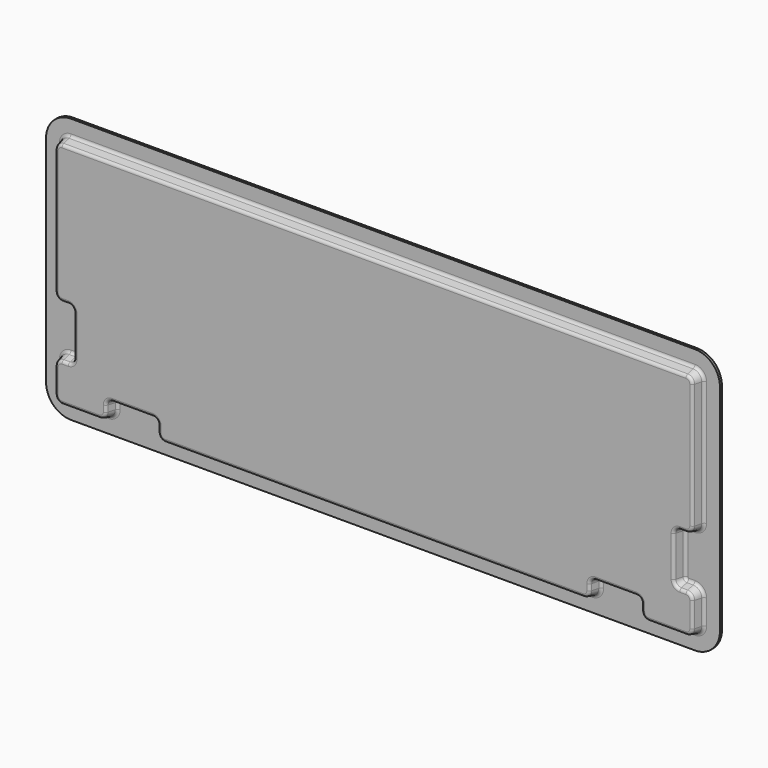
from build123d import *

# Parameters (mm, degrees)
F3_DEPTH = 2
F4_DEPTH = 18
F4_TAPER = -15
F5_R     = 5
F6_T     = 2
F7_DEPTH = 2


# Not quite as in the source:
# - a shell that OpenCascade refuses in one call is made with other operations: the cavity is built on its own and cut out


with BuildPart() as f3:
    # F0 (on Front) → F3 (new body)
    with BuildSketch(Plane.XZ):
        with BuildLine():
            ThreePointArc((540, 172.5), (528.2842712475, 200.7842712475), (500, 212.5))
            Line((500, 212.5), (-500, 212.5))
            ThreePointArc((-500, 212.5), (-528.2842712475, 200.7842712475), (-540, 172.5))
            Line((-540, 172.5), (-540, -172.5))
            ThreePointArc((-540, -172.5), (-528.2842712475, -200.7842712475), (-500, -212.5))
            Line((-500, -212.5), (500, -212.5))
            ThreePointArc((500, -212.5), (528.2842712475, -200.7842712475), (540, -172.5))
            Line((540, -172.5), (540, 172.5))
        make_face()
        with BuildLine():
            ThreePointArc((-525, 172.5), (-517.6776695297, 190.1776695297), (-500, 197.5))
            Line((-500, 197.5), (500, 197.5))
            ThreePointArc((500, 197.5), (517.6776695297, 190.1776695297), (525, 172.5))
            Line((525, 172.5), (525, -172.5))
            ThreePointArc((525, -172.5), (517.6776695297, -190.1776695297), (500, -197.5))
            Line((500, -197.5), (-500, -197.5))
            ThreePointArc((-500, -197.5), (-517.6776695297, -190.1776695297), (-525, -172.5))
            Line((-525, -172.5), (-525, 172.5))
        make_face(mode=Mode.SUBTRACT)
        with BuildLine():
            Line((500, 197.5), (-500, 197.5))
            ThreePointArc((-500, 197.5), (-517.6776695297, 190.1776695297), (-525, 172.5))
            Line((-525, 172.5), (-525, -172.5))
            ThreePointArc((-525, -172.5), (-517.6776695297, -190.1776695297), (-500, -197.5))
            Line((-500, -197.5), (500, -197.5))
            ThreePointArc((500, -197.5), (517.6776695297, -190.1776695297), (525, -172.5))
            Line((525, -172.5), (525, 172.5))
            ThreePointArc((525, 172.5), (517.6776695297, 190.1776695297), (500, 197.5))
        make_face()
    extrude(amount=F3_DEPTH)

    # F2 (on offset) → F4 (join, through all)
    with BuildSketch(Plane.XZ.offset(20)):
        with BuildLine():
            Line((510, -27.5), (510, 172.5))
            ThreePointArc((510, 172.5), (507.0710678119, 179.5710678119), (500, 182.5))
            Line((500, 182.5), (-500, 182.5))
            ThreePointArc((-500, 182.5), (-507.0710678119, 179.5710678119), (-510, 172.5))
            Line((-510, 172.5), (-510, -27.5))
            ThreePointArc((-510, -27.5), (-507.0710678119, -34.5710678119), (-500, -37.5))
            Line((-500, -37.5), (-490, -37.5))
            ThreePointArc((-490, -37.5), (-482.9289321881, -40.4289321881), (-480, -47.5))
            Line((-480, -47.5), (-480, -112.5))
            ThreePointArc((-480, -112.5), (-482.9289321881, -119.5710678119), (-490, -122.5))
            Line((-490, -122.5), (-500, -122.5))
            ThreePointArc((-500, -122.5), (-507.0710678119, -125.4289321881), (-510, -132.5))
            Line((-510, -132.5), (-510, -172.5))
            ThreePointArc((-510, -172.5), (-507.0710678119, -179.5710678119), (-500, -182.5))
            Line((-500, -182.5), (-440, -182.5))
            ThreePointArc((-440, -182.5), (-432.9289321881, -179.5710678119), (-430, -172.5))
            Line((-430, -172.5), (-430, -162.5))
            ThreePointArc((-430, -162.5), (-427.0710678119, -155.4289321881), (-420, -152.5))
            Line((-420, -152.5), (-355, -152.5))
            ThreePointArc((-355, -152.5), (-347.9289321881, -155.4289321881), (-345, -162.5))
            Line((-345, -162.5), (-345, -172.5))
            ThreePointArc((-345, -172.5), (-342.0710678119, -179.5710678119), (-335, -182.5))
            Line((-335, -182.5), (0, -182.5))
            Line((0, -182.5), (335, -182.5))
            ThreePointArc((335, -182.5), (342.0710678119, -179.5710678119), (345, -172.5))
            Line((345, -172.5), (345, -162.5))
            ThreePointArc((345, -162.5), (347.9289321881, -155.4289321881), (355, -152.5))
            Line((355, -152.5), (420, -152.5))
            ThreePointArc((420, -152.5), (427.0710678119, -155.4289321881), (430, -162.5))
            Line((430, -162.5), (430, -172.5))
            ThreePointArc((430, -172.5), (432.9289321881, -179.5710678119), (440, -182.5))
            Line((440, -182.5), (500, -182.5))
            ThreePointArc((500, -182.5), (507.0710678119, -179.5710678119), (510, -172.5))
            Line((510, -172.5), (510, -132.5))
            ThreePointArc((510, -132.5), (507.0710678119, -125.4289321881), (500, -122.5))
            Line((500, -122.5), (490, -122.5))
            ThreePointArc((490, -122.5), (482.9289321881, -119.5710678119), (480, -112.5))
            Line((480, -112.5), (480, -47.5))
            ThreePointArc((480, -47.5), (482.9289321881, -40.4289321881), (490, -37.5))
            Line((490, -37.5), (500, -37.5))
            ThreePointArc((500, -37.5), (507.0710678119, -34.5710678119), (510, -27.5))
        make_face()
    extrude(amount=-F4_DEPTH, taper=F4_TAPER)

    # F5
    f5_edges = [f3.edges().sort_by_distance(p)[0] for p in [
        (427.071068, -20, -155.428932),
        (430, -20, -167.5),
        (432.928932, -20, -179.571068),
        (470, -20, -182.5),
        (507.071068, -20, -179.571068),
        (510, -20, -152.5),
        (507.071068, -20, -125.428932),
        (495, -20, -122.5),
        (482.928932, -20, -119.571068),
        (480, -20, -80),
        (482.928932, -20, -40.428932),
        (495, -20, -37.5),
        (507.071068, -20, -34.571068),
        (510, -20, 72.5),
        (507.071068, -20, 179.571068),
        (0, -20, 182.5),
        (-507.071068, -20, 179.571068),
        (-510, -20, 72.5),
        (-507.071068, -20, -34.571068),
        (-495, -20, -37.5),
        (-482.928932, -20, -40.428932),
        (-480, -20, -80),
        (-482.928932, -20, -119.571068),
        (-495, -20, -122.5),
        (-507.071068, -20, -125.428932),
        (-510, -20, -152.5),
        (-507.071068, -20, -179.571068),
        (-470, -20, -182.5),
        (-432.928932, -20, -179.571068),
        (-430, -20, -167.5),
        (-427.071068, -20, -155.428932),
        (-387.5, -20, -152.5),
        (-347.928932, -20, -155.428932),
        (-345, -20, -167.5),
        (-342.071068, -20, -179.571068),
        (0, -20, -182.5),
        (342.071068, -20, -179.571068),
        (345, -20, -167.5),
        (347.928932, -20, -155.428932),
        (387.5, -20, -152.5),
        (0, -2, -187.323085),
        (423.660631, -2, -158.839369),
        (425.176915, -2, -167.5),
        (429.518496, -2, -182.981504),
        (470, -2, -187.323085),
        (510.481504, -2, -182.981504),
        (514.823085, -2, -152.5),
        (510.481504, -2, -122.018496),
        (495, -2, -117.676915),
        (486.339369, -2, -116.160631),
        (484.823085, -2, -80),
        (486.339369, -2, -43.839369),
        (495, -2, -42.323085),
        (510.481504, -2, -37.981504),
        (514.823085, -2, 72.5),
        (510.481504, -2, 182.981504),
        (0, -2, 187.323085),
        (-510.481504, -2, 182.981504),
        (-514.823085, -2, 72.5),
        (-510.481504, -2, -37.981504),
        (-495, -2, -42.323085),
        (-486.339369, -2, -43.839369),
        (-484.823085, -2, -80),
        (-486.339369, -2, -116.160631),
        (-495, -2, -117.676915),
        (-510.481504, -2, -122.018496),
        (-514.823085, -2, -152.5),
        (-510.481504, -2, -182.981504),
        (-470, -2, -187.323085),
        (-429.518496, -2, -182.981504),
        (-425.176915, -2, -167.5),
        (-423.660631, -2, -158.839369),
        (-387.5, -2, -157.323085),
        (-351.339369, -2, -158.839369),
        (-349.823085, -2, -167.5),
        (-345.481504, -2, -182.981504),
        (345.481504, -2, -182.981504),
        (349.823085, -2, -167.5),
        (351.339369, -2, -158.839369),
        (387.5, -2, -157.323085),
    ]]
    fillet(f5_edges, radius=F5_R)

    # F6: shell of thickness 2, made by hand


with BuildPart() as f6_core1:
    # F6_t2: copy of F3
    add(f3.part)

    # the walls: a layer under each face that stays
    f6_faces = [f6_core1.faces().sort_by_distance(p)[0] for p in [
        (-504, -2, -198.3333333333),
        (0, -3.0332332985, -188.1159132586),
        (-346.0421181596, -3.0332332985, -183.5421181596),
        (346.0421181596, -3.0332332985, -183.5421181596),
        (-350.6159132586, -3.0332332985, -167.5),
        (350.6159132586, -3.0332332985, -167.5),
        (-351.8999827599, -3.0332332985, -159.3999827599),
        (351.8999827599, -3.0332332985, -159.3999827599),
        (-387.5, -3.0332332985, -158.1159132586),
        (387.5, -3.0332332985, -158.1159132586),
        (-423.1000172401, -3.0332332985, -159.3999827599),
        (423.1000172401, -3.0332332985, -159.3999827599),
        (-424.3840867414, -3.0332332985, -167.5),
        (424.3840867414, -3.0332332985, -167.5),
        (-428.9578818404, -3.0332332985, -183.5421181596),
        (428.9578818404, -3.0332332985, -183.5421181596),
        (-470, -3.0332332985, -188.1159132586),
        (470, -3.0332332985, -188.1159132586),
        (-511.0421181596, -3.0332332985, -183.5421181596),
        (511.0421181596, -3.0332332985, -183.5421181596),
        (-515.6159132586, -3.0332332985, -152.5),
        (515.6159132586, -3.0332332985, -152.5),
        (-511.0421173614, -3.0332332985, -121.4578826386),
        (511.0421173614, -3.0332332985, -121.4578826386),
        (-495, -3.0332332985, -116.8840867414),
        (495, -3.0332332985, -116.8840867414),
        (-486.8999825359, -3.0332332985, -115.6000174641),
        (486.8999825359, -3.0332332985, -115.6000174641),
        (-485.6159132586, -3.0332332985, -80),
        (485.6159132586, -3.0332332985, -80),
        (-486.8999827599, -3.0332332985, -44.3999827599),
        (486.8999827599, -3.0332332985, -44.3999827599),
        (-495, -3.0332332985, -43.1159132586),
        (495, -3.0332332985, -43.1159132586),
        (-511.0421181596, -3.0332332985, -38.5421181596),
        (511.0421181596, -3.0332332985, -38.5421181596),
        (-515.6159132586, -3.0332332985, 72.5),
        (515.6159132586, -3.0332332985, 72.5),
        (-511.0421173614, -3.0332332985, 183.5421173614),
        (511.0421173614, -3.0332332985, 183.5421173614),
        (0, -3.0332332985, 188.1159132586),
        (528.2842712475, -1, -200.7842712475),
        (0, -1, -212.5),
        (540, -1, 0),
        (-528.2842712475, -1, -200.7842712475),
        (528.2842712475, -1, 200.7842712475),
        (-540, -1, 0),
        (0, -1, 212.5),
        (-528.2842712475, -1, 200.7842712475),
        (0, -11, -184.9115427319),
        (-343.7762860307, -11, -181.2762860307),
        (343.7762860307, -11, -181.2762860307),
        (-347.4115427319, -11, -167.5),
        (347.4115427319, -11, -167.5),
        (-349.634150407, -11, -157.134150407),
        (349.634150407, -11, -157.134150407),
        (-387.5, -11, -154.9115427319),
        (387.5, -11, -154.9115427319),
        (-425.365849593, -11, -157.134150407),
        (425.365849593, -11, -157.134150407),
        (-427.5884572681, -11, -167.5),
        (427.5884572681, -11, -167.5),
        (-431.2237139693, -11, -181.2762860307),
        (431.2237139693, -11, -181.2762860307),
        (-470, -11, -184.9115427319),
        (470, -11, -184.9115427319),
        (-508.7762860307, -11, -181.2762860307),
        (508.7762860307, -11, -181.2762860307),
        (-512.4115427319, -11, -152.5),
        (512.4115427319, -11, -152.5),
        (-508.7762860307, -11, -123.7237139693),
        (508.7762860307, -11, -123.7237139693),
        (-495, -11, -120.0884572681),
        (495, -11, -120.0884572681),
        (-484.634150407, -11, -117.865849593),
        (484.634150407, -11, -117.865849593),
        (-482.4115427319, -11, -80),
        (482.4115427319, -11, -80),
        (-484.634150407, -11, -42.134150407),
        (484.634150407, -11, -42.134150407),
        (-495, -11, -39.9115427319),
        (495, -11, -39.9115427319),
        (-508.7762860307, -11, -36.2762860307),
        (508.7762860307, -11, -36.2762860307),
        (-512.4115427319, -11, 72.5),
        (512.4115427319, -11, 72.5),
        (-508.7762860307, -11, 181.2762860307),
        (508.7762860307, -11, 181.2762860307),
        (0, -11, 184.9115427319),
        (0, -18.9667667015, -181.7071722051),
        (-341.5104539018, -18.9667667015, -179.0104539018),
        (341.5104534312, -18.9667667015, -179.0104534312),
        (-344.2071722051, -18.9667667015, -167.5),
        (344.2071722051, -18.9667667015, -167.5),
        (-347.3683182781, -18.9667667015, -154.8683182781),
        (347.3683182781, -18.9667667015, -154.8683182781),
        (-387.5, -18.9667667015, -151.7071722051),
        (387.5, -18.9667667015, -151.7071722051),
        (-427.6316817219, -18.9667667015, -154.8683182781),
        (427.6316817219, -18.9667667015, -154.8683182781),
        (-430.7928277949, -18.9667667015, -167.5),
        (430.7928277949, -18.9667667015, -167.5),
        (-433.4895460982, -18.9667667015, -179.0104539018),
        (433.4895460982, -18.9667667015, -179.0104539018),
        (-470, -18.9667667015, -181.7071722051),
        (470, -18.9667667015, -181.7071722051),
        (-506.5104539018, -18.9667667015, -179.0104539018),
        (506.5104539018, -18.9667667015, -179.0104539018),
        (-509.2071722051, -18.9667667015, -152.5),
        (509.2071722051, -18.9667667015, -152.5),
        (-506.5104539018, -18.9667667015, -125.9895460982),
        (506.5104539018, -18.9667667015, -125.9895460982),
        (-495, -18.9667667015, -123.2928277949),
        (495, -18.9667667015, -123.2928277949),
        (-482.3683182781, -18.9667667015, -120.1316817219),
        (482.3683182781, -18.9667667015, -120.1316817219),
        (-479.2071722051, -18.9667667015, -80),
        (479.2071722051, -18.9667667015, -80),
        (-482.3683182781, -18.9667667015, -39.8683182781),
        (482.3683188297, -18.9667667015, -39.8683188297),
        (-495, -18.9667667015, -36.7071722051),
        (495, -18.9667667015, -36.7071722051),
        (-506.5104539018, -18.9667667015, -34.0104539018),
        (506.5104534312, -18.9667667015, -34.0104534312),
        (-509.2071722051, -18.9667667015, 72.5),
        (509.2071722051, -18.9667667015, 72.5),
        (-506.5104539018, -18.9667667015, 179.0104539018),
        (506.5104539018, -18.9667667015, 179.0104539018),
        (0, -18.9667667015, 181.7071722051),
        (0, -20, 0),
    ]]
    thicken(f6_faces, amount=-F6_T, mode=Mode.SUBTRACT)


with BuildPart() as f3_1:
    add(f3.part)

    # what is left inside the walls is the cavity
    f6_cavity = [f6_core1.part.solids().sort_by_distance(p)[0] for p in [
        (0, -0.02, -63.719907),
    ]]
    add(f6_cavity, mode=Mode.SUBTRACT)


with BuildPart() as f7:
    # F0 (on Front) → F7 (new body)
    with BuildSketch(Plane.XZ):
        with BuildLine():
            ThreePointArc((540, 172.5), (528.2842712475, 200.7842712475), (500, 212.5))
            Line((500, 212.5), (-500, 212.5))
            ThreePointArc((-500, 212.5), (-528.2842712475, 200.7842712475), (-540, 172.5))
            Line((-540, 172.5), (-540, -172.5))
            ThreePointArc((-540, -172.5), (-528.2842712475, -200.7842712475), (-500, -212.5))
            Line((-500, -212.5), (500, -212.5))
            ThreePointArc((500, -212.5), (528.2842712475, -200.7842712475), (540, -172.5))
            Line((540, -172.5), (540, 172.5))
        make_face()
        with BuildLine():
            ThreePointArc((-525, 172.5), (-517.6776695297, 190.1776695297), (-500, 197.5))
            Line((-500, 197.5), (500, 197.5))
            ThreePointArc((500, 197.5), (517.6776695297, 190.1776695297), (525, 172.5))
            Line((525, 172.5), (525, -172.5))
            ThreePointArc((525, -172.5), (517.6776695297, -190.1776695297), (500, -197.5))
            Line((500, -197.5), (-500, -197.5))
            ThreePointArc((-500, -197.5), (-517.6776695297, -190.1776695297), (-525, -172.5))
            Line((-525, -172.5), (-525, 172.5))
        make_face(mode=Mode.SUBTRACT)
        with BuildLine():
            Line((500, 197.5), (-500, 197.5))
            ThreePointArc((-500, 197.5), (-517.6776695297, 190.1776695297), (-525, 172.5))
            Line((-525, 172.5), (-525, -172.5))
            ThreePointArc((-525, -172.5), (-517.6776695297, -190.1776695297), (-500, -197.5))
            Line((-500, -197.5), (500, -197.5))
            ThreePointArc((500, -197.5), (517.6776695297, -190.1776695297), (525, -172.5))
            Line((525, -172.5), (525, 172.5))
            ThreePointArc((525, 172.5), (517.6776695297, 190.1776695297), (500, 197.5))
        make_face()
    extrude(amount=-F7_DEPTH)


solid = Compound([f3_1.part, f7.part])
